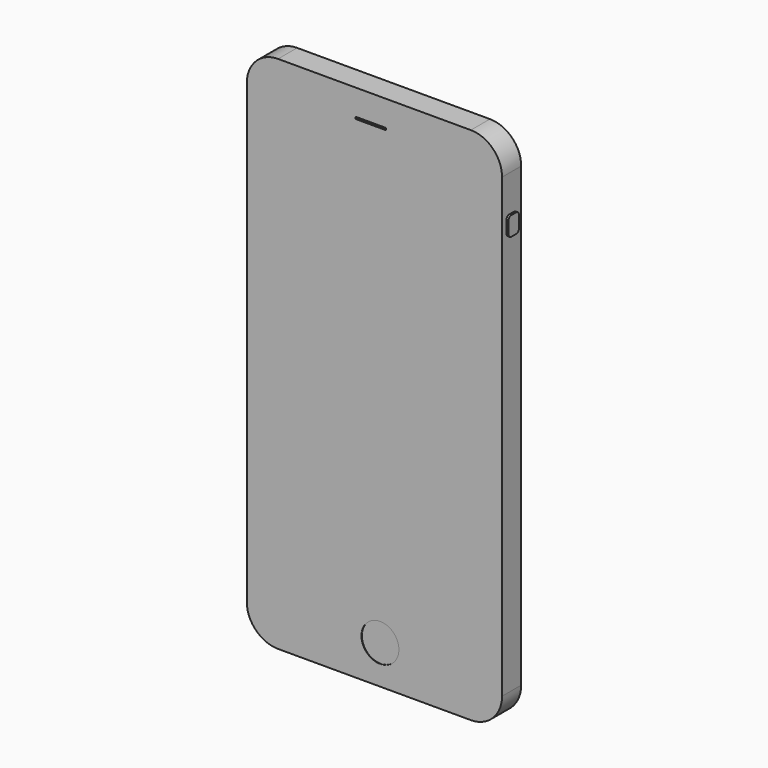
from build123d import *

# Parameters (mm, degrees)
F0_W         = 77.8764
F0_H         = 158.496
F1_DEPTH     = 7.2898
F2_R         = 9.525
F3_R         = 5.7077755574
F4_DEPTH     = 0.127
F5_W         = 9.2544863001
F5_H         = 0.6169676781
F6_DEPTH     = 0.381
F8_DEPTH     = 0.635
F9_R         = 1.016
F10_R        = 1.9930126565
F11_DEPTH    = 12.7
F13_W        = 8.6497310549
F13_H        = 2.2564521059
F14_DEPTH    = 12.7
F16_DEPTH    = 2.159
F18_DEPTH    = 0.635
F19_T1_DEPTH = 2.8833260431
F19_T3_DEPTH = 2.8575
F19_T5_DEPTH = 2.8319706152
F21_DEPTH    = 0.635
F22_T1_DEPTH = 3.4834715988
F22_T3_DEPTH = 3.4925
F22_T5_DEPTH = 3.5015570173
F23_R        = 0.635


# Not quite as in the source:
# - a fillet or chamfer that OpenCascade refuses, or shapes differently, is made with other operations: its cross-section is extruded or revolved along the edge and cut away or added


with BuildPart() as f1:
    # F0 (on Front) → F1 (new body)
    with BuildSketch(Plane.XZ):
        with Locations((-10.9280409528, 4.5388489962)):
            Rectangle(F0_W, F0_H)
    extrude(amount=F1_DEPTH)

    # F2
    f2_edges = [f1.edges().sort_by_distance(p)[0] for p in [
        (-49.866241, -3.6449, 83.786849),
        (28.010159, -3.6449, 83.786849),
        (28.010159, -3.6449, -74.709151),
        (-49.866241, -3.6449, -74.709151),
    ]]
    fillet(f2_edges, radius=F2_R)

    # F3 (on face) → F4 (cut)
    with BuildSketch(Plane.XZ.offset(7.2898)):
        with Locations((-9.174161778, -62.8947635373)):
            Circle(F3_R)
    extrude(amount=-F4_DEPTH, mode=Mode.SUBTRACT)

    # F5 (on face) → F6 (cut)
    with BuildSketch(Plane.XZ.offset(7.2898)):
        with Locations((-12.0077328756, 75.6440907717)):
            Rectangle(F5_W, F5_H)
    extrude(amount=-F6_DEPTH, mode=Mode.SUBTRACT)

    # F7 (on face) → F8 (join)
    with BuildSketch(Plane.YZ.offset(28.0101590472)):
        Polygon((-1.6678672982, 63.1312280893), (-5.6040398777, 63.1312280893), (-5.5761812255, 57.3286004364), (-1.6678672982, 57.3286004364), align=None)
    extrude(amount=F8_DEPTH)

    # F9
    f9_edges = [f1.edges().sort_by_distance(p)[0] for p in [
        (28.327659, -5.60404, 63.131228),
        (28.327659, -5.576181, 57.3286),
        (28.327659, -1.667867, 63.131228),
        (28.327659, -1.667867, 57.3286),
    ]]
    fillet(f9_edges, radius=F9_R)

    # F10 (on face) → F11 (cut)
    with BuildSketch(Plane(origin=(0, 0, -74.7091510038), x_dir=(1, 0, 0), z_dir=(0, 0, -1))):
        with Locations((-36.9087584466, 4.1701743638)):
            Circle(F10_R)
    extrude(amount=-F11_DEPTH, mode=Mode.SUBTRACT)

    # F13 (on face) → F14 (cut)
    with BuildSketch(Plane(origin=(0, 0, -74.7091510038), x_dir=(1, 0, 0), z_dir=(0, 0, -1))):
        with Locations((-8.9176273905, 3.8671875373)):
            Rectangle(F13_W, F13_H)
    extrude(amount=-F14_DEPTH, mode=Mode.SUBTRACT)

    # F15 (on face) → F16 (cut)
    with BuildSketch(Plane(origin=(-49.8662409528, 0, 0), x_dir=(0, -1, 0), z_dir=(-1, 0, 0))):
        Polygon((1.5233993763, 64.8115798831), (1.6149281291, 56.9802224636), (5.1021506079, 56.9802224636), (5.1021506079, 64.8115798831), align=None)
    extrude(amount=-F16_DEPTH, mode=Mode.SUBTRACT)

    # F17 (on face) → F18 (join)
    with BuildSketch(Plane(origin=(-49.8662409528, 0, 0), x_dir=(0, -1, 0), z_dir=(-1, 0, 0))):
        Polygon((2.3726914078, 50.4039227962), (2.4461376015, 44.0468862653), (4.1652750224, 44.0468862653), (4.1652750224, 50.4039227962), align=None)
    extrude(amount=F18_DEPTH)

    # F19: fillet of radius 0.889 on 4 edges, made by hand

    # F19_s2 → F19_t1 (cut)
    with BuildSketch(Plane.YZ.offset(-52.7495669959)):
        with BuildLine():
            ThreePointArc((-3.272021825, 50.4039227962), (-2.639783189, 50.1398990415), (-2.3830811527, 49.5046523961))
            Line((-2.3830811527, 49.5046523961), (-2.3726914078, 50.4039227962))
            Line((-2.3726914078, 50.4039227962), (-3.272021825, 50.4039227962))
        make_face()
    extrude(amount=F19_T1_DEPTH, mode=Mode.SUBTRACT)

    # F19_s4 → F19_t3 (cut)
    with BuildSketch(Plane.YZ.offset(-52.7237409528)):
        with BuildLine():
            ThreePointArc((-3.2762750224, 50.4039227962), (-3.9048929509, 50.1435407247), (-4.1652750224, 49.5149227962))
            Line((-4.1652750224, 49.5149227962), (-4.1652750224, 50.4039227962))
            Line((-4.1652750224, 50.4039227962), (-3.2762750224, 50.4039227962))
        make_face()
        with BuildLine():
            ThreePointArc((-4.1652750224, 44.9358862653), (-3.9048929509, 44.3072683368), (-3.2762750224, 44.0468862653))
            Line((-3.2762750224, 44.0468862653), (-4.1652750224, 44.0468862653))
            Line((-4.1652750224, 44.0468862653), (-4.1652750224, 44.9358862653))
        make_face()
    extrude(amount=F19_T3_DEPTH, mode=Mode.SUBTRACT)

    # F19_s6 → F19_t5 (cut)
    with BuildSketch(Plane.YZ.offset(-52.698211568)):
        with BuildLine():
            ThreePointArc((-3.3249258476, 44.0468862653), (-2.6999496023, 44.3036476293), (-2.4359851753, 44.9256158651))
            Line((-2.4359851753, 44.9256158651), (-2.4461376015, 44.0468862653))
            Line((-2.4461376015, 44.0468862653), (-3.3249258476, 44.0468862653))
        make_face()
    extrude(amount=F19_T5_DEPTH, mode=Mode.SUBTRACT)

    # F20 (on face) → F21 (join)
    with BuildSketch(Plane(origin=(-49.8662409528, 0, 0), x_dir=(0, -1, 0), z_dir=(-1, 0, 0))):
        Polygon((2.1069913637, 41.4195619524), (2.087448258, 35.2439321578), (3.8858172484, 35.2439321578), (3.8858172484, 41.4195619524), align=None)
    extrude(amount=F21_DEPTH)

    # F22: fillet of radius 1.143 on 4 edges, made by hand

    # F22_s2 → F22_t1 (cut)
    with BuildSketch(Plane.YZ.offset(-53.3497125516)):
        with BuildLine():
            ThreePointArc((-3.2463800032, 41.4195619524), (-2.4394367914, 41.0860628189), (-2.1033857264, 40.2801790179))
            Line((-2.1033857264, 40.2801790179), (-2.1069913637, 41.4195619524))
            Line((-2.1069913637, 41.4195619524), (-3.2463800032, 41.4195619524))
        make_face()
    extrude(amount=F22_T1_DEPTH, mode=Mode.SUBTRACT)

    # F22_s4 → F22_t3 (cut)
    with BuildSketch(Plane.YZ.offset(-53.3587409528)):
        with BuildLine():
            ThreePointArc((-2.7428172484, 41.4195619524), (-3.5510402993, 41.0847850032), (-3.8858172484, 40.2765619524))
            Line((-3.8858172484, 40.2765619524), (-3.8858172484, 41.4195619524))
            Line((-3.8858172484, 41.4195619524), (-2.7428172484, 41.4195619524))
        make_face()
        with BuildLine():
            ThreePointArc((-3.8858172484, 36.3869321578), (-3.5510402993, 35.5787091069), (-2.7428172484, 35.2439321578))
            Line((-2.7428172484, 35.2439321578), (-3.8858172484, 35.2439321578))
            Line((-3.8858172484, 35.2439321578), (-3.8858172484, 36.3869321578))
        make_face()
    extrude(amount=F22_T3_DEPTH, mode=Mode.SUBTRACT)

    # F22_s6 → F22_t5 (cut)
    with BuildSketch(Plane.YZ.offset(-53.3677979701)):
        with BuildLine():
            ThreePointArc((-3.2340710649, 35.2439321578), (-2.4245701983, 35.579988946), (-2.091076788, 36.3905492233))
            Line((-2.091076788, 36.3905492233), (-2.087448258, 35.2439321578))
            Line((-2.087448258, 35.2439321578), (-3.2340710649, 35.2439321578))
        make_face()
    extrude(amount=F22_T5_DEPTH, mode=Mode.SUBTRACT)

    # F23
    f23_edges = [f1.edges().sort_by_distance(p)[0] for p in [
        (-47.707241, -1.569164, 60.895901),
        (-47.707241, -3.358539, 56.980222),
        (-47.707241, -5.102151, 60.895901),
        (-47.707241, -3.312775, 64.81158),
        (-49.866241, -1.569164, 60.895901),
        (-48.786741, -5.102151, 56.980222),
        (-48.786741, -1.523399, 64.81158),
        (-49.866241, -5.102151, 60.895901),
        (-49.866241, -3.312775, 64.81158),
        (-49.866241, -3.358539, 56.980222),
    ]]
    fillet(f23_edges, radius=F23_R)


solid = f1.part
